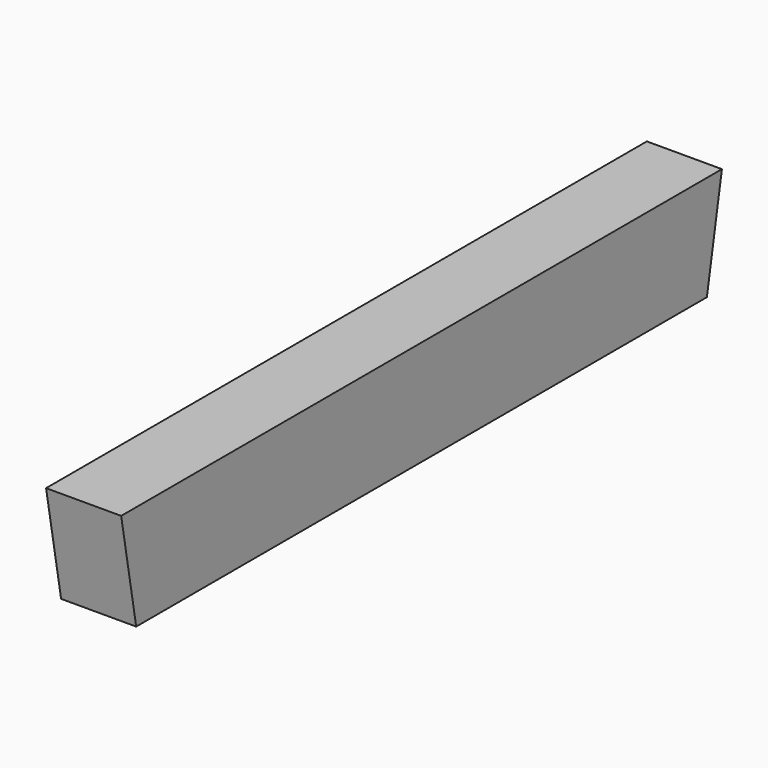
from build123d import *

# Parameters (mm, degrees)
F0_W     = 20
F0_H     = 28
F1_DEPTH = 200
F2_SIZE2 = 27.99999
F2_SIZE  = 4.99999
F3_SIZE2 = 4.99999
F3_SIZE  = 27.99999


# Not quite as in the source:
# - a fillet or chamfer is up to 0.001 mm smaller than in the source, because OpenCascade refuses the exact size


with BuildPart() as f1:
    # F0 (on Front) → F1 (new body)
    with BuildSketch(Plane.XZ):
        Rectangle(F0_W, F0_H)
    extrude(amount=F1_DEPTH)

    # F2 (size 5 and 28 in the source; OpenCascade refuses exactly that, so slightly less here)
    f2_edges = [f1.edges().sort_by_distance(p)[0] for p in [
        (0, -200, -14),
    ]]
    f2_side = f1.faces().sort_by_distance((0, -100, -14))[0]
    chamfer(f2_edges, length=F2_SIZE, length2=F2_SIZE2, reference=f2_side)

    # F3 (size 28 and 5 in the source; OpenCascade refuses exactly that, so slightly less here)
    f3_edges = [f1.edges().sort_by_distance(p)[0] for p in [
        (0, 0, -14),
    ]]
    f3_side = f1.faces().sort_by_distance((0, 0, 0))[0]
    chamfer(f3_edges, length=F3_SIZE, length2=F3_SIZE2, reference=f3_side)


solid = f1.part
